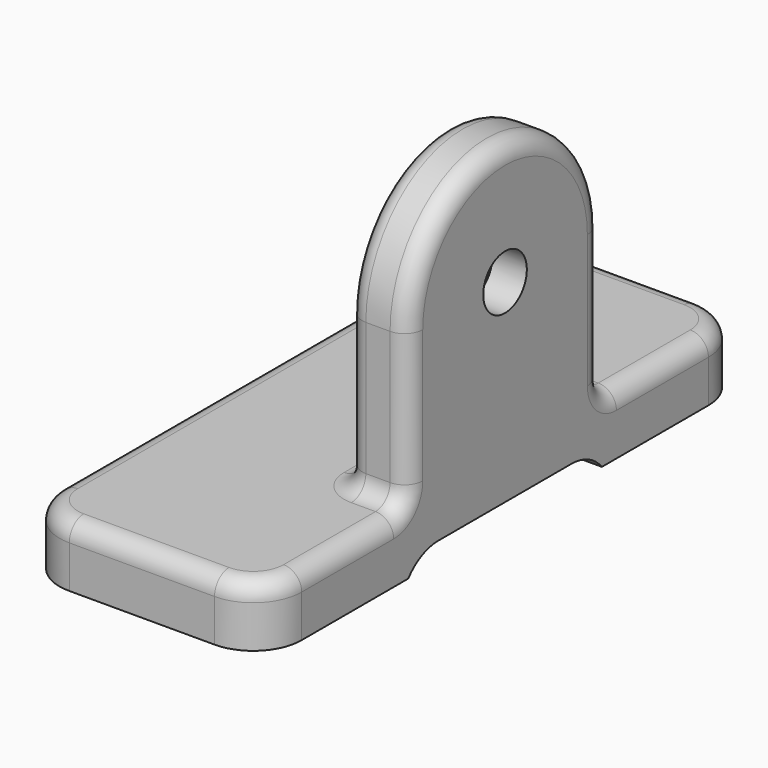
from build123d import *

# Parameters (mm, degrees)
F0_W          = 40
F0_H          = 100
F1_DEPTH      = 10
F3_DEPTH      = 10
F4_W          = 40
F4_H          = 3
F5_DEPTH      = 40.001
F6_R          = 2.25
F7_DEPTH      = 40.001
F8_R          = 4.5
F9_DEPTH      = 5.7
F10_T1_DEPTH  = 40
F10_T3_DEPTH  = 40
F10_T5_DEPTH  = 50
F10_T7_DEPTH  = 50
F10_T9_DEPTH  = 50
F10_T11_DEPTH = 50
F11_R         = 3


# Not quite as in the source:
# - a fillet or chamfer that OpenCascade refuses, or shapes differently, is made with other operations: its cross-section is extruded or revolved along the edge and cut away or added


with BuildPart() as f1:
    # F0 (on Top) → F1 (new body)
    with BuildSketch(Plane.XY):
        with Locations((20, 50)):
            Rectangle(F0_W, F0_H)
    extrude(amount=F1_DEPTH)

    # F2 (on face) → F3 (join)
    with BuildSketch(Plane.YZ.offset(40)):
        with BuildLine():
            Line((30, 35), (30, 0))
            Line((30, 0), (70, 0))
            Line((70, 0), (70, 35))
            ThreePointArc((70, 35), (50, 55), (30, 35))
        make_face()
    extrude(amount=-F3_DEPTH)

    # F4 (on face) → F5 (cut, through all)
    with BuildSketch(Plane.YZ.offset(40)):
        with Locations((50, 1.5)):
            Rectangle(F4_W, F4_H)
    extrude(amount=-F5_DEPTH, mode=Mode.SUBTRACT)

    # F6 (on face) → F7 (cut, through all)
    with BuildSketch(Plane.YZ.offset(40)):
        with Locations((50, 35)):
            Circle(F6_R)
    extrude(amount=-F7_DEPTH, mode=Mode.SUBTRACT)

    # F8 (on face) → F9 (cut)
    with BuildSketch(Plane.YZ.offset(40)):
        with Locations((50, 35)):
            Circle(F8_R)
    extrude(amount=-F9_DEPTH, mode=Mode.SUBTRACT)

    # F10: fillet of radius 8 on 6 edges, made by hand

    # F10_s2 → F10_t1 (join)
    with BuildSketch(Plane.YZ):
        with BuildLine():
            ThreePointArc((70, 0), (67.2191036167, 2.2111025509), (63.7550020016, 3))
            Line((63.7550020016, 3), (70, 3))
            Line((70, 3), (70, 0))
        make_face()
    extrude(amount=F10_T1_DEPTH)

    # F10_s4 → F10_t3 (join)
    with BuildSketch(Plane.YZ):
        with BuildLine():
            ThreePointArc((36.2449979984, 3), (32.7808963833, 2.2111025509), (30, 0))
            Line((30, 0), (30, 3))
            Line((30, 3), (36.2449979984, 3))
        make_face()
    extrude(amount=F10_T3_DEPTH)

    # F10_s6 → F10_t5 (cut)
    with BuildSketch(Plane.XY.offset(-20)):
        with BuildLine():
            ThreePointArc((0, 8), (2.3431457505, 2.3431457505), (8, 0))
            Line((8, 0), (0, 0))
            Line((0, 0), (0, 8))
        make_face()
    extrude(amount=F10_T5_DEPTH, mode=Mode.SUBTRACT)

    # F10_s8 → F10_t7 (cut)
    with BuildSketch(Plane.XY.offset(-20)):
        with BuildLine():
            ThreePointArc((0, 92), (2.3431457505, 97.6568542495), (8, 100))
            Line((8, 100), (0, 100))
            Line((0, 100), (0, 92))
        make_face()
    extrude(amount=F10_T7_DEPTH, mode=Mode.SUBTRACT)

    # F10_s10 → F10_t9 (cut)
    with BuildSketch(Plane.XY.offset(-20)):
        with BuildLine():
            ThreePointArc((40, 8), (37.6568542495, 2.3431457505), (32, 0))
            Line((32, 0), (40, 0))
            Line((40, 0), (40, 8))
        make_face()
    extrude(amount=F10_T9_DEPTH, mode=Mode.SUBTRACT)

    # F10_s12 → F10_t11 (cut)
    with BuildSketch(Plane.XY.offset(-20)):
        with BuildLine():
            ThreePointArc((40, 92), (37.6568542495, 97.6568542495), (32, 100))
            Line((32, 100), (40, 100))
            Line((40, 100), (40, 92))
        make_face()
    extrude(amount=F10_T11_DEPTH, mode=Mode.SUBTRACT)

    # F11
    f11_edges = [f1.edges().sort_by_distance(p)[0] for p in [
        (40, 50, 55),
        (30, 50, 55),
        (35, 70, 10),
        (35, 30, 10),
        (0, 50, 10),
        (2.343146, 2.343146, 10),
        (30, 50, 10),
        (40, 19, 10),
        (37.656854, 2.343146, 10),
        (20, 0, 10),
        (2.343146, 97.656854, 10),
        (20, 100, 10),
        (37.656854, 97.656854, 10),
        (40, 81, 10),
        (40, 70, 22.5),
        (40, 30, 22.5),
        (30, 70, 22.5),
        (30, 30, 22.5),
    ]]
    fillet(f11_edges, radius=F11_R)


solid = f1.part
